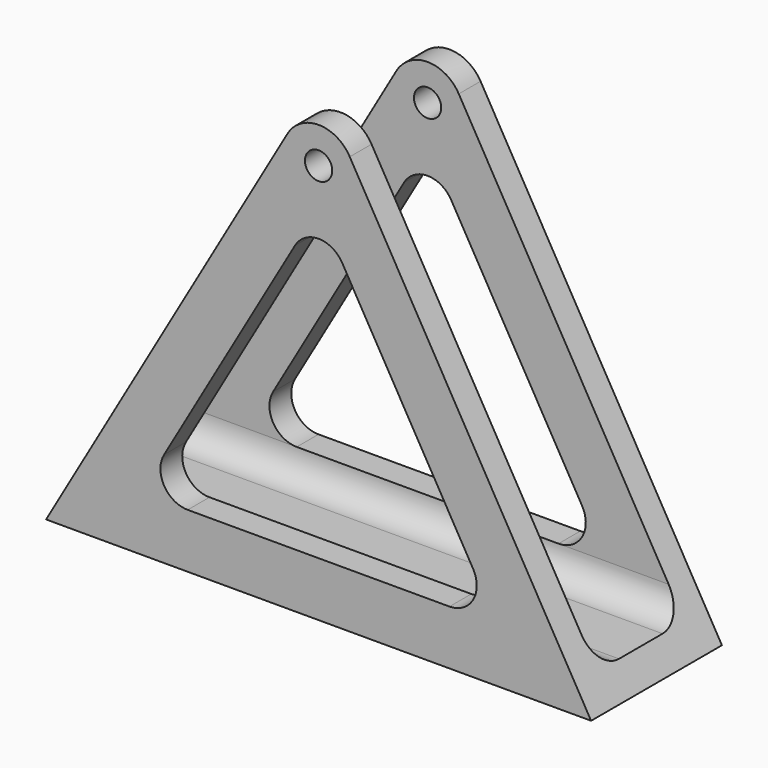
from build123d import *

# Parameters (mm, degrees)
F0_R     = 3.175
F1_DEPTH = 38.1
F3_W     = 127
F3_H     = 25.4
F4_DEPTH = 95.251
F6_DEPTH = 38.101
F7_R     = 6.35
F8_R     = 6.34999


# Not quite as in the source:
# - a fillet or chamfer is up to 0.001 mm smaller than in the source, because OpenCascade refuses the exact size


with BuildPart() as f1:
    # F0 (on Front) → F1 (new body)
    with BuildSketch(Plane.XZ):
        with BuildLine():
            Line((-49.5749215348, 67.2876468139), (-105.8131025593, -30.1197400458))
            Line((-105.8131025593, -30.1197400458), (21.1868974407, -30.1197400458))
            Line((21.1868974407, -30.1197400458), (-35.0512835838, 67.2876468139))
            ThreePointArc((-35.0512835838, 67.2876468139), (-42.3131025593, 71.4802599542), (-49.5749215348, 67.2876468139))
        make_face()
        with Locations((-42.3131025593, 63.0950336736)):
            Circle(F0_R, mode=Mode.SUBTRACT)
    extrude(amount=F1_DEPTH)

    # F3 (on offset) → F4 (cut, through all)
    with BuildSketch(Plane(origin=(0, 0, -23.7697400458), x_dir=(1, 0, 0), z_dir=(0, 0, -1))):
        with Locations((-42.3131025593, 19.05)):
            Rectangle(F3_W, F3_H)
    extrude(amount=-F4_DEPTH, mode=Mode.SUBTRACT)

    # F5 (on face) → F6 (cut, through all)
    with BuildSketch(Plane.XZ.offset(38.1)):
        Polygon((-0.8101478154, -17.4197400458), (-42.3131025593, 54.4654862348), (-83.8160573032, -17.4197400458), align=None)
    extrude(amount=-F6_DEPTH, mode=Mode.SUBTRACT)

    # F7
    f7_edges = [f1.edges().sort_by_distance(p)[0] for p in [
        (-42.313103, -34.925, 54.465486),
        (-83.816057, -34.925, -17.41974),
        (-0.810148, -34.925, -17.41974),
        (-0.810148, -3.175, -17.41974),
        (-83.816057, -3.175, -17.41974),
        (-42.313103, -3.175, 54.465486),
    ]]
    fillet(f7_edges, radius=F7_R)

    # F8 (radius 6.35 in the source; OpenCascade refuses exactly that, so slightly less here)
    f8_edges = [f1.edges().sort_by_distance(p)[0] for p in [
        (-42.313103, -6.35, -23.76974),
        (-42.313103, -31.75, -23.76974),
    ]]
    fillet(f8_edges, radius=F8_R)


solid = f1.part
